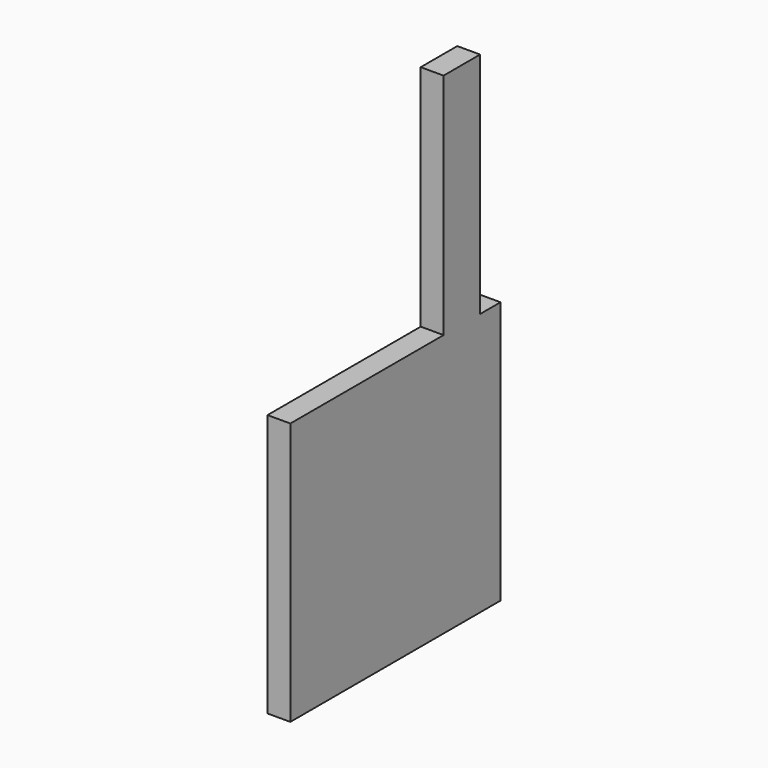
from build123d import *

# Parameters (mm, degrees)
F1_DEPTH = 1


# Not quite as in the source:
# - a feature names something its author has since deleted; it is built from what else it names


with BuildPart() as f1:
    # F0 (on Right) → F1 (new body)
    with BuildSketch(Plane.YZ):
        Polygon((8.384144865, 0), (0, 0), (0, -11.5), (11.5, -11.5), (11.5, 0), (10.384144865, 0), (10.384144865, 10), (8.384144865, 10), align=None)
    extrude(amount=F1_DEPTH)


solid = f1.part
